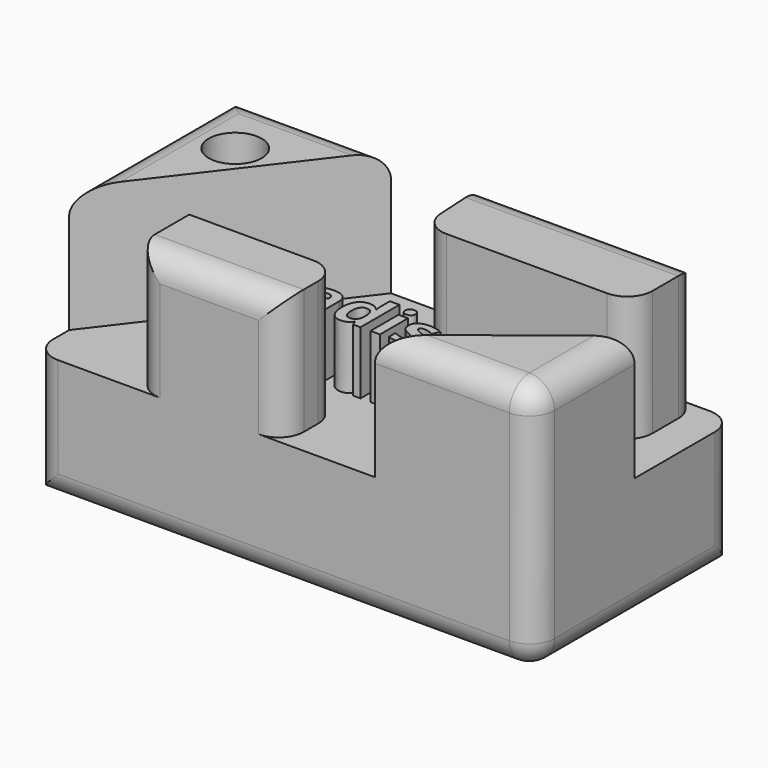
from build123d import *

# Parameters (mm, degrees)
F0_W         = 50.8
F0_H         = 12.7
F1_DEPTH     = 25.4
F2_W         = 15.1013697773
F2_H         = 6.9062042326
F3_DEPTH     = 12.7
F4_R         = 2.54
F5_TEXT_SIZE = 6.4890521268
F6_DEPTH     = 6.35
F7_R         = 2.6871571871
F8_DEPTH     = 25.4


# Not quite as in the source:
# - Text() gives the source's letters only with a copy of the font that has no kerning and outlines rounded to 1/6400 em; it was checked with that copy


with BuildPart() as f1:
    # F0 (on Front) → F1 (new body)
    with BuildSketch(Plane.XZ):
        with Locations((25.4, 6.35)):
            Rectangle(F0_W, F0_H)
    extrude(amount=F1_DEPTH)

    # F2 (on face) → F3 (join)
    with BuildSketch(Plane.XY.offset(12.7)):
        Polygon((0, 0), (0, -20.8298545331), (15.944538638, 0), align=None)
        Polygon((47.0943748951, 0), (25.4, 0), (25.8735474199, -8.3708763123), (47.0943748951, -8.3708763123), align=None)
        Polygon((50.8, -12.7), (34.634437412, -25.4), (50.8, -25.4), align=None)
        with Locations((17.8493151113, -21.9468978837)):
            Rectangle(F2_W, F2_H)
    extrude(amount=F3_DEPTH)

    # F4
    f4_edges = [f1.edges().sort_by_distance(p)[0] for p in [
        (0, -10.414927, 25.4),
        (7.972269, 0, 25.4),
        (36.247187, 0, 25.4),
        (17.849315, -25.4, 25.4),
        (42.717219, -25.4, 25.4),
        (50.8, -19.05, 25.4),
        (50.8, -12.7, 0),
        (25.4, -25.4, 0),
        (50.8, -25.4, 12.7),
        (50.8, 0, 6.35),
        (0, -25.4, 6.35),
        (47.094375, 0, 19.05),
        (25.4, -25.4, 19.05),
        (10.29863, -25.4, 19.05),
        (47.094375, -8.370876, 19.05),
        (25.873547, -8.370876, 19.05),
        (25.4, -18.493796, 19.05),
    ]]
    fillet(f4_edges, radius=F4_R)

    # F5 (on face) → F6 (join)
    with BuildSketch(Plane.XY.offset(12.7)):
        with Locations((11.6802919656, -15.5737223104)):
            Text('Madison', F5_TEXT_SIZE, font='Open Sans', font_style=FontStyle.BOLD, text_align=(TextAlign.LEFT, TextAlign.BOTTOM))
    extrude(amount=F6_DEPTH)

    # F7 (on face) → F8 (cut)
    with BuildSketch(Plane.XY.offset(25.4)):
        with Locations((6.0530682708, -7.3585202089)):
            Circle(F7_R)
    extrude(amount=-F8_DEPTH, mode=Mode.SUBTRACT)


solid = f1.part
